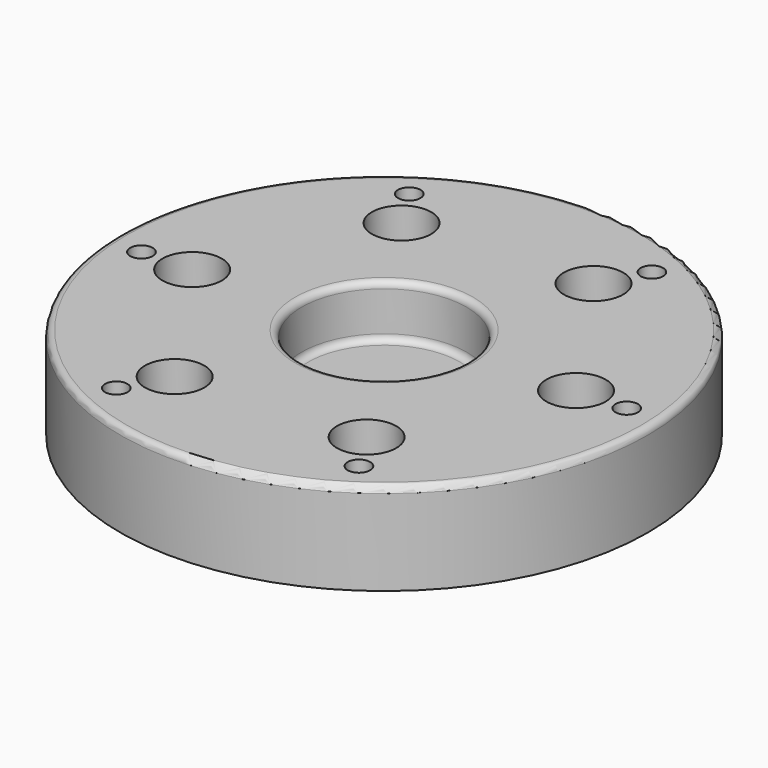
from build123d import *

# Parameters (mm, degrees)
F0_R      = 40
F0_R_2    = 1.7
F1_DEPTH  = 14
F2_R      = 4.5
F2_R_2    = 1.7
F3_DEPTH  = 7
F4_R      = 4.5
F4_R_2    = 1.7
F5_DEPTH  = 4.6
F6_R      = 12.5
F7_DEPTH  = 8
F8_R      = 1
F10_R     = 32.1563127089
F11_DEPTH = 0.3


with BuildPart() as f1:
    # F0 (on Top) → F1 (new body)
    with BuildSketch(Plane.XY):
        Circle(F0_R)
        with Locations((-15.4640459878, -31.3984598617)):
            Circle(F0_R_2, mode=Mode.SUBTRACT)
        with Locations((-11.9054035877, -24.7893397535)):
            Circle(F0_R_2, mode=Mode.SUBTRACT)
        with Locations((-34.9238868738, -2.3069732602)):
            Circle(F0_R_2, mode=Mode.SUBTRACT)
        with Locations((-27.4208997634, -2.0842879275)):
            Circle(F0_R_2, mode=Mode.SUBTRACT)
        with Locations((19.4598408861, -29.0914866016)):
            Circle(F0_R_2, mode=Mode.SUBTRACT)
        with Locations((15.5154961757, -22.705051826)):
            Circle(F0_R_2, mode=Mode.SUBTRACT)
        with Locations((-15.5154961757, 22.705051826)):
            Circle(F0_R_2, mode=Mode.SUBTRACT)
        with Locations((-19.4598408861, 29.0914866016)):
            Circle(F0_R_2, mode=Mode.SUBTRACT)
        with Locations((27.4208997634, 2.0842879275)):
            Circle(F0_R_2, mode=Mode.SUBTRACT)
        with Locations((34.9238868738, 2.3069732602)):
            Circle(F0_R_2, mode=Mode.SUBTRACT)
        with Locations((11.9054035877, 24.7893397535)):
            Circle(F0_R_2, mode=Mode.SUBTRACT)
        with Locations((15.4640459878, 31.3984598617)):
            Circle(F0_R_2, mode=Mode.SUBTRACT)
    extrude(amount=F1_DEPTH)

    # F2 (on face) → F3 (cut)
    with BuildSketch(Plane.XY.offset(14)):
        with Locations((-15.5154961757, 22.705051826)):
            Circle(F2_R)
        with Locations((-15.5154961757, 22.705051826)):
            Circle(F2_R_2, mode=Mode.SUBTRACT)
        with Locations((-27.4208997634, -2.0842879275)):
            Circle(F2_R)
        with Locations((-27.4208997634, -2.0842879275)):
            Circle(F2_R_2, mode=Mode.SUBTRACT)
        with Locations((-11.9054035877, -24.7893397535)):
            Circle(F2_R)
        with Locations((-11.9054035877, -24.7893397535)):
            Circle(F2_R_2, mode=Mode.SUBTRACT)
        with Locations((15.5154961757, -22.705051826)):
            Circle(F2_R)
        with Locations((15.5154961757, -22.705051826)):
            Circle(F2_R_2, mode=Mode.SUBTRACT)
        with Locations((27.4208997634, 2.0842879275)):
            Circle(F2_R)
        with Locations((27.4208997634, 2.0842879275)):
            Circle(F2_R_2, mode=Mode.SUBTRACT)
        with Locations((11.9054035877, 24.7893397535)):
            Circle(F2_R)
        with Locations((11.9054035877, 24.7893397535)):
            Circle(F2_R_2, mode=Mode.SUBTRACT)
    extrude(amount=-F3_DEPTH, mode=Mode.SUBTRACT)

    # F4 (on face) → F5 (cut)
    with BuildSketch(Plane(origin=(0, 0, 0), x_dir=(1, 0, 0), z_dir=(0, 0, -1))):
        with Locations((27.4208997634, -2.0842879275)):
            Circle(F4_R)
        with Locations((27.4208997634, -2.0842879275)):
            Circle(F4_R_2, mode=Mode.SUBTRACT)
        with Locations((15.5154961757, 22.705051826)):
            Circle(F4_R)
        with Locations((15.5154961757, 22.705051826)):
            Circle(F4_R_2, mode=Mode.SUBTRACT)
        with Locations((-11.9054035877, 24.7893397535)):
            Circle(F4_R)
        with Locations((-11.9054035877, 24.7893397535)):
            Circle(F4_R_2, mode=Mode.SUBTRACT)
        with Locations((-27.4208997634, 2.0842879275)):
            Circle(F4_R)
        with Locations((-27.4208997634, 2.0842879275)):
            Circle(F4_R_2, mode=Mode.SUBTRACT)
        with Locations((-15.5154961757, -22.705051826)):
            Circle(F4_R)
        with Locations((-15.5154961757, -22.705051826)):
            Circle(F4_R_2, mode=Mode.SUBTRACT)
        with Locations((11.9054035877, -24.7893397535)):
            Circle(F4_R)
        with Locations((11.9054035877, -24.7893397535)):
            Circle(F4_R_2, mode=Mode.SUBTRACT)
        with Locations((27.4208997634, -2.0842879275)):
            Circle(F4_R_2)
    extrude(amount=-F5_DEPTH, mode=Mode.SUBTRACT)

    # F6 (on face) → F7 (cut)
    with BuildSketch(Plane.XY.offset(14)):
        Circle(F6_R)
    extrude(amount=-F7_DEPTH, mode=Mode.SUBTRACT)

    # F8
    f8_edges = [f1.edges().sort_by_distance(p)[0] for p in [
        (-12.5, 0, 6),
        (-12.5, 0, 14),
        (-40, 0, 14),
    ]]
    fillet(f8_edges, radius=F8_R)

    # F10 (on offset) → F11 (join)
    with BuildSketch(Plane(origin=(0, 0, 4.6), x_dir=(1, 0, 0), z_dir=(0, 0, -1))):
        Circle(F10_R)
    extrude(amount=-F11_DEPTH)


solid = f1.part
